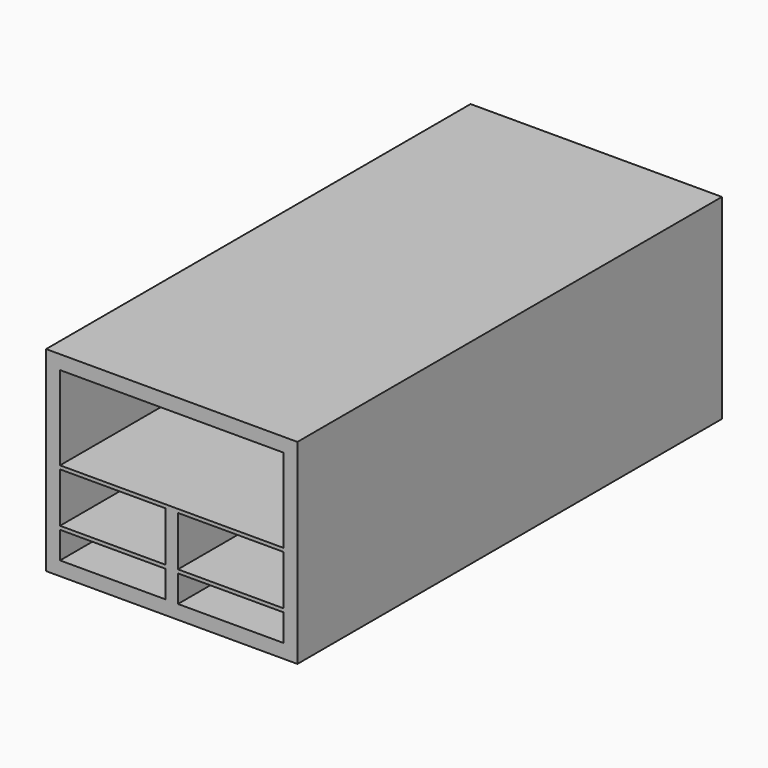
from build123d import *

# Parameters (mm, degrees)
F1_DEPTH = 190
F0_W     = 80
F0_H     = 30.028
F0_W_2   = 35.56
F0_H_2   = 17.78
F0_H_3   = 9.652
F0_W_3   = 2.22
F2_DEPTH = 5


with BuildPart() as f1:
    # F0 (on Front) → F1 (new body)
    with BuildSketch(Plane.XZ):
        Polygon((45, 30), (45, 35), (-40, 35), (-40, 30.452), (-40, 30), (40, 30), align=None)
        Polygon((-40, 30.452), (-40, 35), (-45, 35), (-45, -30), (-40, -30), (-40, -20.348), (-40, -19.078), (-40, -1.298), (-40, -0.028), (-40, 30), align=None)
        Polygon((45, -30), (45, 30), (40, 30), (40, -0.028), (40, -1.298), (40, -19.078), (40, -20.348), (40, -30), align=None)
        Polygon((45, -35), (45, -30), (40, -30), (4.44, -30), (2.22, -30), (-2.22, -30), (-4.44, -30), (-40, -30), (-45, -30), (-45, -35), align=None)
        Polygon((40, -1.298), (40, -0.028), (-40, -0.028), (-40, -1.298), (-4.44, -1.298), (-2.22, -1.298), (2.22, -1.298), (4.44, -1.298), align=None)
        Polygon((4.44, -20.348), (40, -20.348), (40, -19.078), (4.44, -19.078), (2.22, -19.078), (2.22, -20.348), align=None)
        Polygon((-40, -19.078), (-40, -20.348), (-4.44, -20.348), (-2.22, -20.348), (-2.22, -19.078), (-4.44, -19.078), align=None)
        Polygon((-2.22, -30), (2.22, -30), (2.22, -20.348), (2.22, -19.078), (2.22, -1.298), (-2.22, -1.298), (-2.22, -19.078), (-2.22, -20.348), align=None)
    extrude(amount=F1_DEPTH)

    # F0 (on Front) → F2 (join)
    with BuildSketch(Plane.XZ):
        with Locations((0, 14.986)):
            Rectangle(F0_W, F0_H)
        with Locations((-22.22, -10.188)):
            Rectangle(F0_W_2, F0_H_2)
        with Locations((22.22, -10.188)):
            Rectangle(F0_W_2, F0_H_2)
        with Locations((22.22, -25.174)):
            Rectangle(F0_W_2, F0_H_3)
        with Locations((-22.22, -25.174)):
            Rectangle(F0_W_2, F0_H_3)
        with Locations((-3.33, -10.188)):
            Rectangle(F0_W_3, F0_H_2)
        with Locations((-3.33, -25.174)):
            Rectangle(F0_W_3, F0_H_3)
        with Locations((3.33, -25.174)):
            Rectangle(F0_W_3, F0_H_3)
        with Locations((3.33, -10.188)):
            Rectangle(F0_W_3, F0_H_2)
    extrude(amount=F2_DEPTH)


solid = f1.part
